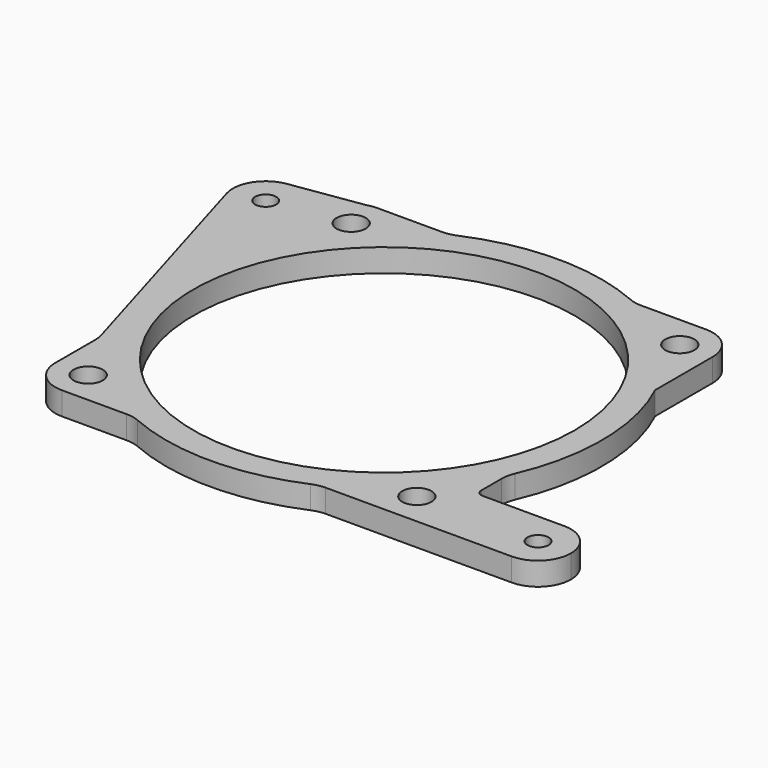
from build123d import *

# Parameters (mm, degrees)
F0_R     = 2.22
F0_R_2   = 29
F0_R_3   = 1.6
F2_DEPTH = 3.5
F3_R     = 4.375
F3_R_2   = 2.22
F4_DEPTH = 1


with BuildPart() as f2:
    # F0 (on Top) → F2 (new body)
    with BuildSketch(Plane.XY):
        with BuildLine():
            Line((-28.0399272842, 48.7993610323), (-26.564868493, 49.0218929201))
            ThreePointArc((-26.564868493, 49.0218929201), (-27.3107436298, 48.965946953), (-28.0399272842, 48.7993610323))
        make_face()
        with BuildLine():
            Line((-16.69420754, 49.0218929201), (-26.564868493, 49.0218929201))
            Line((-26.564868493, 49.0218929201), (-28.0399272842, 48.7993610323))
            Line((-28.0399272842, 48.7993610323), (-38.8670578152, 47.165946953))
            ThreePointArc((-38.8670578152, 47.165946953), (-42.3386518344, 44.9075872285), (-42.9166986895, 40.8066098434))
            Line((-42.9166986895, 40.8066098434), (-31.7693524819, 3.0351716781))
            ThreePointArc((-31.7693524819, 3.0351716781), (-31.6162535325, 2.3348780924), (-31.564868493, 1.6198886013))
            Line((-31.564868493, 1.6198886013), (-31.564868493, -5.9781070799))
            ThreePointArc((-31.564868493, -5.9781070799), (-30.1004023989, -9.5136409858), (-26.564868493, -10.9781070799))
            Line((-26.564868493, -10.9781070799), (-16.69420754, -10.9781070799))
            ThreePointArc((-16.69420754, -10.9781070799), (-15.6812440963, -11.0817916221), (-14.7102921129, -11.3885450552))
            ThreePointArc((-14.7102921129, -11.3885450552), (-1.564868493, -14.1081070799), (11.5805551269, -11.3885450552))
            ThreePointArc((11.5805551269, -11.3885450552), (12.5515071103, -11.0817916221), (13.564470554, -10.9781070799))
            Line((13.564470554, -10.9781070799), (23.435131507, -10.9781070799))
            Line((23.435131507, -10.9781070799), (41.8588173216, -10.9781070799))
            ThreePointArc((41.8588173216, -10.9781070799), (39.4580409401, -10.3640246311), (37.6469744143, -8.6726161862))
            ThreePointArc((37.6469744143, -8.6726161862), (37.5867252108, -8.5760349073), (37.5286903027, -8.4781070799))
            ThreePointArc((37.5286903027, -8.4781070799), (37.5286903027, -3.4781070799), (41.8588173216, -0.9781070799))
            Line((41.8588173216, -0.9781070799), (29.435131507, -0.9781070799))
            ThreePointArc((29.435131507, -0.9781070799), (28.7280247258, -0.6852138611), (28.435131507, 0.0218929201))
            Line((28.435131507, 0.0218929201), (28.435131507, 3.8925538731))
            ThreePointArc((28.435131507, 3.8925538731), (28.5388160493, 4.9055173169), (28.8455694823, 5.8764693002))
            ThreePointArc((28.8455694823, 5.8764693002), (31.5613609993, 19.521712514), (28.435131507, 33.0788093672))
            Line((28.435131507, 33.0788093672), (28.435131507, 44.0218929201))
            ThreePointArc((28.435131507, 44.0218929201), (26.9706654129, 47.5574268261), (23.435131507, 49.0218929201))
            Line((23.435131507, 49.0218929201), (13.564470554, 49.0218929201))
            ThreePointArc((13.564470554, 49.0218929201), (12.5515071103, 49.1255774624), (11.5805551269, 49.4323308955))
            ThreePointArc((11.5805551269, 49.4323308955), (-1.564868493, 52.1518929201), (-14.7102921129, 49.4323308955))
            ThreePointArc((-14.7102921129, 49.4323308955), (-15.6812440963, 49.1255774624), (-16.69420754, 49.0218929201))
        make_face()
        with Locations((-26.5610932079, -5.9743317948)):
            Circle(F0_R, mode=Mode.SUBTRACT)
        with Locations((23.4313562219, -5.9743317948)):
            Circle(F0_R, mode=Mode.SUBTRACT)
        with Locations((-1.564868493, 19.0218929201)):
            Circle(F0_R_2, mode=Mode.SUBTRACT)
        with Locations((-38.1211826784, 42.2218929201)):
            Circle(F0_R_3, mode=Mode.SUBTRACT)
        with Locations((-26.561093208, 44.0181176351)):
            Circle(F0_R, mode=Mode.SUBTRACT)
        with BuildLine():
            ThreePointArc((25.6513562219, 44.0181176351), (24.2809134408, 41.9671050725), (21.8615791662, 42.4483405824))
            ThreePointArc((21.8615791662, 42.4483405824), (22.5817990031, 46.0691301977), (25.6513562219, 44.0181176351))
        make_face(mode=Mode.SUBTRACT)
        with BuildLine():
            ThreePointArc((46.8588173216, -5.9781070799), (45.3943512276, -2.4425731739), (41.8588173216, -0.9781070799))
            ThreePointArc((41.8588173216, -0.9781070799), (37.5286903027, -3.4781070799), (37.5286903027, -8.4781070799))
            ThreePointArc((37.5286903027, -8.4781070799), (37.5867252108, -8.5760349073), (37.6469744143, -8.6726161862))
            ThreePointArc((37.6469744143, -8.6726161862), (39.4580409401, -10.3640246311), (41.8588173216, -10.9781070799))
            ThreePointArc((41.8588173216, -10.9781070799), (45.3943512276, -9.5136409858), (46.8588173216, -5.9781070799))
        make_face()
        with Locations((41.8588173216, -5.9781070799)):
            Circle(F0_R_3, mode=Mode.SUBTRACT)
    extrude(amount=F2_DEPTH)

    # F3 (on face) → F4 (cut)
    with BuildSketch(Plane(origin=(0, 0, 0), x_dir=(1, 0, 0), z_dir=(0, 0, -1))):
        with Locations((23.4313562219, 5.9743317948)):
            Circle(F3_R)
        with Locations((23.4313562219, 5.9743317948)):
            Circle(F3_R_2, mode=Mode.SUBTRACT)
        with Locations((-26.5610932079, 5.9743317948)):
            Circle(F3_R)
        with Locations((-26.5610932079, 5.9743317948)):
            Circle(F3_R_2, mode=Mode.SUBTRACT)
        with Locations((-26.561093208, -44.0181176351)):
            Circle(F3_R)
        with Locations((-26.561093208, -44.0181176351)):
            Circle(F3_R_2, mode=Mode.SUBTRACT)
        with Locations((23.4313562219, -44.0181176351)):
            Circle(F3_R)
        with Locations((23.4313562219, -44.0181176351)):
            Circle(F3_R_2, mode=Mode.SUBTRACT)
        with Locations((-26.5610932079, 5.9743317948)):
            Circle(F3_R_2)
        with Locations((23.4313562219, 5.9743317948)):
            Circle(F3_R_2)
        with Locations((23.4313562219, -44.0181176351)):
            Circle(F3_R_2)
        with Locations((-26.561093208, -44.0181176351)):
            Circle(F3_R_2)
    extrude(amount=-F4_DEPTH, mode=Mode.SUBTRACT)


solid = f2.part
